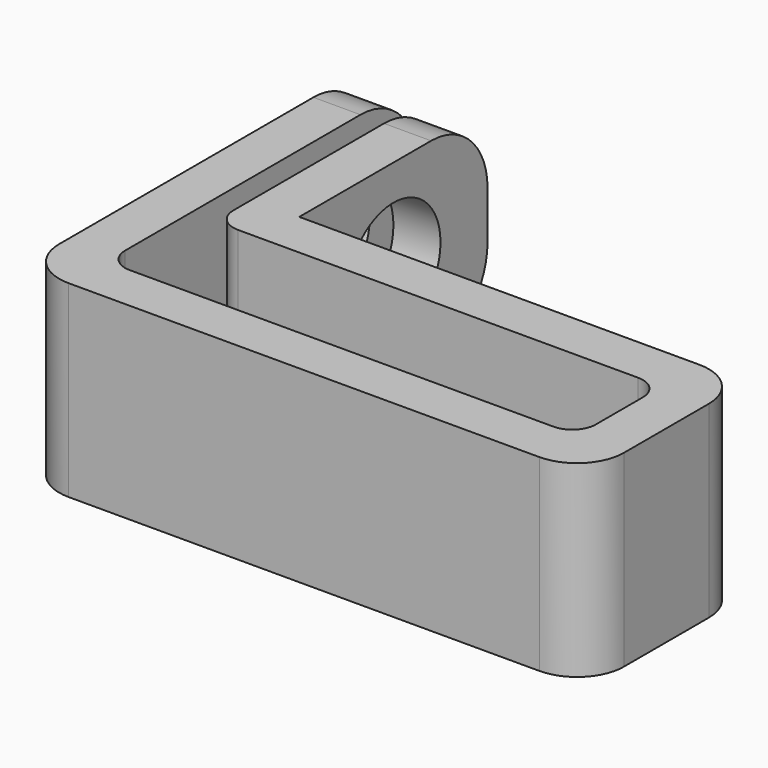
from build123d import *

# Parameters (mm, degrees)
F1_DEPTH = 8
F3_R     = 3
F2_R     = 2.5
F4_DEPTH = 5.001
F5_R     = 2
F6_R     = 1


# Not quite as in the source:
# - a feature names something its author has since deleted; it is built from what else it names


with BuildPart() as f1:
    # F0 (on Top) → F1 (new body)
    with BuildSketch(Plane.XY):
        Polygon((0, 0), (0, 16.5), (-2, 16.5), (-2, -2), (22, -2), (22, 6.5), (3, 6.5), (3, 16.5), (1, 16.5), (1, 4.5), (20, 4.5), (20, 0), align=None)
    extrude(amount=-F1_DEPTH)

    # F3
    f3_edges = [f1.edges().sort_by_distance(p)[0] for p in [
        (-1, 16.5, 0),
        (-1, 16.5, -8),
        (2, 16.5, 0),
        (2, 16.5, -8),
    ]]
    fillet(f3_edges, radius=F3_R)

    # F2 (on face) → F4 (cut, through all)
    with BuildSketch(Plane.YZ.offset(3)):
        with Locations((11.5, -4)):
            Circle(F2_R)
    extrude(amount=-F4_DEPTH, mode=Mode.SUBTRACT)

    # F5
    f5_edges = [f1.edges().sort_by_distance(p)[0] for p in [
        (22, 6.5, -4),
        (22, -2, -4),
        (-2, -2, -4),
    ]]
    fillet(f5_edges, radius=F5_R)

    # F6
    f6_edges = [f1.edges().sort_by_distance(p)[0] for p in [
        (20, 4.5, -4),
        (20, 0, -4),
        (0, 0, -4),
        (1, 4.5, -4),
    ]]
    fillet(f6_edges, radius=F6_R)


solid = f1.part
